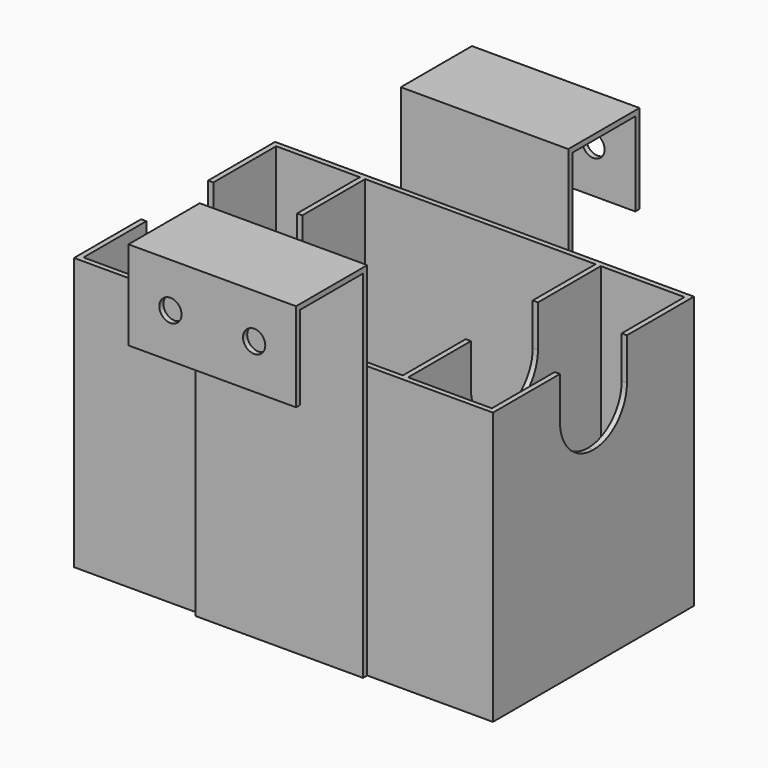
from build123d import *

# Parameters (mm, degrees)
F0_W      = 127
F0_H      = 76.2
F1_DEPTH  = 82.55
F3_W      = 25.4
F3_H      = 73.025
F3_W_2    = 69.85
F4_DEPTH  = 80.9625
F6_DEPTH  = 127.001
F8_DEPTH  = 1.5875
F10_DEPTH = 1.5875
F11_W     = 50.8
F11_H     = 26.9875
F11_H_2   = 1.5875
F11_H_3   = 25.4
F12_DEPTH = 1.5875
F13_W     = 50.8
F13_H     = 1.5875
F14_DEPTH = 25.4
F15_R     = 3.3734375
F16_DEPTH = 1.5875
F17_R     = 3.3734375
F18_DEPTH = 1.5875


# Not quite as in the source:
# - a length typed as a fraction of an inch, garbled in the dataset ("3 / 203.2 mm" for 3/8 in), is restored


with BuildPart() as f1:
    # F0 (on Top) → F1 (new body)
    with BuildSketch(Plane.XY):
        Rectangle(F0_W, F0_H)
    extrude(amount=F1_DEPTH)

    # F3 (on face) → F4 (cut)
    with BuildSketch(Plane.XY.offset(82.55)):
        Polygon((-61.9125, 36.5125), (-61.9125, 0), (-61.9125, -36.5125), (-36.5125, -36.5125), (-36.5125, 36.5125), align=None)
        with Locations((49.2125, 0)):
            Rectangle(F3_W, F3_H)
        Rectangle(F3_W_2, F3_H)
    extrude(amount=-F4_DEPTH, mode=Mode.SUBTRACT)

    # F5 (on face) → F6 (cut, through all)
    with BuildSketch(Plane.YZ.offset(63.5)):
        with BuildLine():
            Line((12.7, 69.85), (12.7, 82.55))
            Line((12.7, 82.55), (0, 82.55))
            Line((0, 82.55), (-12.7, 82.55))
            Line((-12.7, 82.55), (-12.7, 69.85))
            ThreePointArc((-12.7, 69.85), (-8.9802561211, 60.8697438789), (0, 57.15))
            ThreePointArc((0, 57.15), (8.9802561211, 60.8697438789), (12.7, 69.85))
        make_face()
    extrude(amount=-F6_DEPTH, mode=Mode.SUBTRACT)

    # F7 (on face) → F8 (join)
    with BuildSketch(Plane.XZ.offset(38.1)):
        Polygon((-12.7, 0), (0, 0), (12.7, 0), (25.4, 0), (25.4, 107.95), (12.7, 107.95), (-12.7, 107.95), (-25.4, 107.95), (-25.4, 0), align=None)
    extrude(amount=F8_DEPTH)

    # F9 (on face) → F10 (join)
    with BuildSketch(Plane(origin=(0, 38.1, 0), x_dir=(-1, 0, 0), z_dir=(0, 1, 0))):
        Polygon((-12.7, 0), (0, 0), (12.7, 0), (25.4, 0), (25.4, 82.55), (-25.4, 82.55), (-25.4, 0), align=None)
        Polygon((-25.4, 82.55), (25.4, 82.55), (25.4, 107.95), (12.7, 107.95), (-12.7, 107.95), (-25.4, 107.95), align=None)
    extrude(amount=F10_DEPTH)

    # F11 (on face) → F12 (join)
    with BuildSketch(Plane.XY.offset(107.95)):
        with Locations((0, -51.59375)):
            Rectangle(F11_W, F11_H)
        with Locations((0, 38.89375)):
            Rectangle(F11_W, F11_H_2)
        with Locations((0, 52.3875)):
            Rectangle(F11_W, F11_H_3)
    extrude(amount=F12_DEPTH)

    # F13 (on face) → F14 (join)
    with BuildSketch(Plane(origin=(0, 0, 107.95), x_dir=(1, 0, 0), z_dir=(0, 0, -1))):
        with Locations((0, 64.29375)):
            Rectangle(F13_W, F13_H)
        with Locations((0, -64.29375)):
            Rectangle(F13_W, F13_H)
    extrude(amount=F14_DEPTH)

    # F15 (on face) → F16 (cut)
    with BuildSketch(Plane.XZ.offset(65.0875)):
        with Locations((12.7, 96.04375)):
            Circle(F15_R)
        with Locations((-12.7, 96.04375)):
            Circle(F15_R)
    extrude(amount=-F16_DEPTH, mode=Mode.SUBTRACT)

    # F17 (on face) → F18 (cut)
    with BuildSketch(Plane(origin=(0, 65.0875, 0), x_dir=(-1, 0, 0), z_dir=(0, 1, 0))):
        with Locations((12.7, 96.04375)):
            Circle(F17_R)
        with Locations((-12.7, 96.04375)):
            Circle(F17_R)
    extrude(amount=-F18_DEPTH, mode=Mode.SUBTRACT)


solid = f1.part
